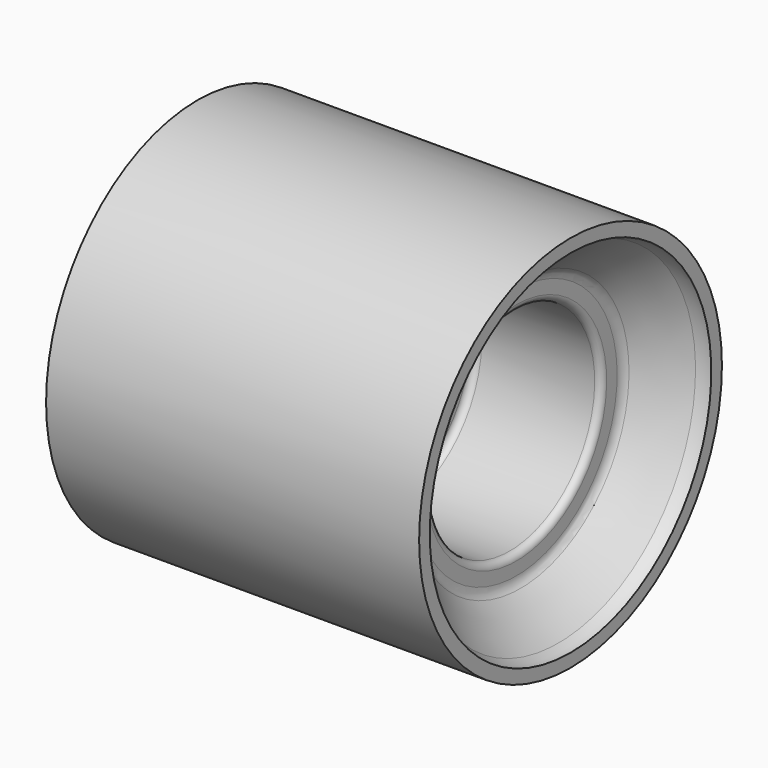
from build123d import *


with BuildPart() as f1:
    # F0 (on Front) → F1 (revolve)
    with BuildSketch(Plane.XZ):
        with BuildLine():
            Line((46.6274327665, 20.4293505417), (52.3332152067, 25.8130880211))
            add(Edge.make_bspline(
                [(52.3332152067, 25.8130880211), (52.6873531533, 26.0396653478), (53.287973728, 26.3773534836), (53.9061448765, 26.4795545854), (54.1609440093, 26.4919212472)],
                knots=[0.0753740232, 0.0753740232, 0.0753740232, 0.0753740232, 0.236653892, 0.3473965491, 0.3473965491, 0.3473965491, 0.3473965491], degree=3))
            Line((54.1609440093, 26.4919212472), (54.1609440093, 28.4919212472))
            Line((54.1609440093, 28.4919212472), (0, 28.4919212472))
            Line((0, 28.4919212472), (-2, 28.4919212472))
            Line((-2, 28.4919212472), (-2, 0))
            Line((-2, 0), (0, 0))
            Line((0, 0), (0, 12.5))
            Line((0, 12.5), (26, 12.5))
            ThreePointArc((26, 12.5), (26.7071067812, 12.7928932188), (27, 13.5))
            Line((27, 13.5), (27, 15))
            ThreePointArc((27, 15), (27.2928932188, 15.7071067812), (28, 16))
            Line((28, 16), (44.9999994072, 16))
            ThreePointArc((44.9999994072, 16), (45.707106398, 16.2928934284), (45.9999994072, 17.0000005928))
            Line((45.9999994072, 17.0000005928), (45.9999982367, 18.9746813235))
            ThreePointArc((45.9999982367, 18.9746813235), (46.1635437461, 19.7667886958), (46.6274327665, 20.4293505417))
        make_face()
    revolve(axis=Axis((19.5, 0, 0), (-1, 0, 0)))


solid = f1.part
